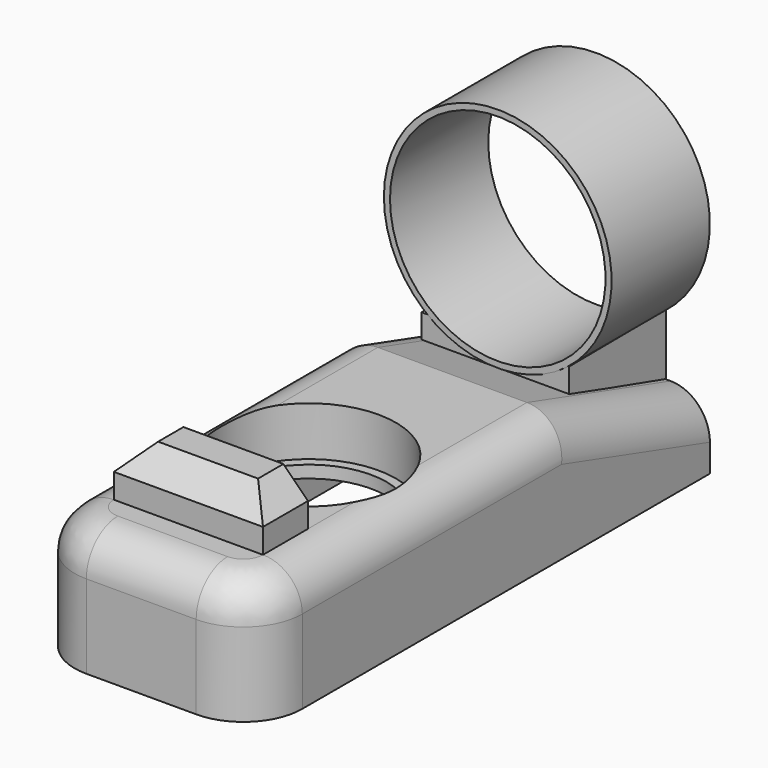
from build123d import *

# Parameters (mm, degrees)
F0_W           = 46.3467240334
F0_H           = 115.6897172332
F1_DEPTH       = 25
F2_R           = 12
F4_DEPTH       = 40
F4_DEPTH_BACK  = 40
F6_R           = 17.7712313218
F7_DEPTH       = 10
F8_R           = 23.1733620167
F9_DEPTH       = 25
F11_R          = 21.9307918762
F12_DEPTH      = 25
F14_DEPTH      = 15
F14_DEPTH_BACK = 15
F15_T          = 2.5
F16_R          = 15.8642477534
F17_DEPTH      = 25
F18_DEPTH      = 5
F19_DEPTH      = 25
F20_T1_DEPTH   = 101.1275982577
F20_T3_DEPTH   = 92.184276345
F20_T5_DEPTH   = 22.3467240334
F20_T8_ANGLE   = 90
F20_T12_DEPTH  = 92.184276345
F20_T17_DEPTH  = 92.184276345
F20_T22_DEPTH  = 92.184276345
F20_T27_DEPTH  = 101.1275982577
F20_T30_ANGLE  = 90
F21_W          = 30.3467240334
F21_H          = 11.4395302832
F22_DEPTH      = 10
F23_SIZE       = 5


# Not quite as in the source:
# - a fillet or chamfer that OpenCascade refuses, or shapes differently, is made with other operations: its cross-section is extruded or revolved along the edge and cut away or added
# - a shell that OpenCascade refuses in one call is made with other operations: the cavity is built on its own and cut out


with BuildPart() as f1:
    # F0 (on Top) → F1 (new body)
    with BuildSketch(Plane.XY):
        with Locations((7.814258337, 1.8636099994)):
            Rectangle(F0_W, F0_H)
    extrude(amount=F1_DEPTH)

    # F2
    f2_edges = [f1.edges().sort_by_distance(p)[0] for p in [
        (30.98762, -55.981249, 12.5),
        (-15.359104, -55.981249, 12.5),
    ]]
    fillet(f2_edges, radius=F2_R)

    # F3 (on Right) → F4 (cut, two sides)
    with BuildSketch(Plane.YZ) as f4_sk:
        Polygon((0, 31.970962882), (68.2880878448, 11.4047080278), (67.6364898682, 28.4685865045), align=None)
    extrude(amount=F4_DEPTH, mode=Mode.SUBTRACT)
    extrude(f4_sk.sketch, amount=-F4_DEPTH_BACK, mode=Mode.SUBTRACT)


with BuildPart() as f1_1:
    # F5: moved
    add(f1.part.moved(Location((-7.1676671505, 0, 0))))

    # F6 (on face) → F7 (cut)
    with BuildSketch(Plane.XY.offset(25)):
        with Locations((0, -12.5934332609)):
            Circle(F6_R)
    extrude(amount=-F7_DEPTH, mode=Mode.SUBTRACT)

    # F15: shell of thickness 2.5, made by hand


with BuildPart() as f9:
    # F8 (on face) → F9 (new body)
    with BuildSketch(Plane(origin=(0, 59.708468616, 0), x_dir=(-1, 0, 0), z_dir=(0, 1, 0))):
        with Locations((-0.6465911865, 33.9257717133)):
            Circle(F8_R)
    extrude(amount=-F9_DEPTH)


with BuildPart() as f9_1:
    # F10: moved
    add(f9.part.moved(Location((0, 0, 10.7776373625))))

    # F11 (on face) → F12 (cut)
    with BuildSketch(Plane(origin=(0, 59.708468616, 0), x_dir=(-1, 0, 0), z_dir=(0, 1, 0))):
        with Locations((-0.6465911865, 44.7034090757)):
            Circle(F11_R)
    extrude(amount=-F12_DEPTH, mode=Mode.SUBTRACT)


with BuildPart() as f14:
    # F13 (on Right) → F14 (new body, two sides)
    with BuildSketch(Plane.YZ) as f14_sk:
        Polygon((59.624966234, 14.1331925988), (59.624966234, 21.5853508562), (34.9215567112, 21.3780961931), align=None)
    extrude(amount=F14_DEPTH)
    extrude(f14_sk.sketch, amount=-F14_DEPTH_BACK)


with BuildPart() as f15_core1:
    # F15_t2: copy of F1
    add(f1_1.part)

    # the walls: a layer under each face that stays
    f15_faces = [f15_core1.faces().sort_by_distance(p)[0] for p in [
        (-22.5267708302, 7.8636099994, 12.5),
        (-19.0120522044, -52.4665299914, 12.5),
        (-14.8023168246, -42.7933155742, 25),
        (0.6465911865, 41.4274091283, 19.4943116685),
        (0.6465911865, 59.708468616, 6.9943116685),
        (0.6465911865, -55.9812486172, 12.5),
        (23.8199532032, 7.8636099994, 12.5),
        (20.3052345774, -52.4665299914, 12.5),
        (-17.7712313218, -12.5934332609, 20),
        (0, -12.5934332609, 15),
    ]]
    thicken(f15_faces, amount=-F15_T, mode=Mode.SUBTRACT)

    # F15_s3 → F15_t4 (revolve, cut)
    with BuildSketch(Plane.XZ.offset(12.5934332609)):
        Polygon((17.7462313218, 15.025), (20.2712313218, 15), (20.2712313218, 12.5), (17.7712313218, 12.5), align=None)
    revolve(axis=Axis((0, -12.5934332609, 15), (0, 0, 1)), mode=Mode.SUBTRACT)


with BuildPart() as f1_2:
    add(f1_1.part)

    # what is left inside the walls is the cavity
    f15_cavity = [f15_core1.part.solids().sort_by_distance(p)[0] for p in [
        (0.646591, -16.584676, 0.025),
    ]]
    add(f15_cavity, mode=Mode.SUBTRACT)

    # F16 (on face) → F17 (cut)
    with BuildSketch(Plane.XY.offset(15)):
        with Locations((0, -12.5934332609)):
            Circle(F16_R)
    extrude(amount=-F17_DEPTH, mode=Mode.SUBTRACT)

    # F18 (add): a face of the model
    f18_faces = [f14.part.faces().sort_by_distance(p)[0] for p in [
        (0, 47.2732614726, 21.4817235246),
    ]]

    add(f9_1.part)  # F18 merges F9

    add(f14.part)  # F18 merges F14
    extrude(f18_faces, amount=F18_DEPTH)

    # F11 (on face) → F19 (cut)
    with BuildSketch(Plane(origin=(0, 59.708468616, 0), x_dir=(-1, 0, 0), z_dir=(0, 1, 0))):
        with Locations((-0.6465911865, 44.7034090757)):
            Circle(F11_R)
    extrude(amount=-F19_DEPTH, mode=Mode.SUBTRACT)

    # F20: fillet of radius 8 on 7 edges, made by hand

    # F20_s2 → F20_t1 (cut)
    with BuildSketch(Plane.XZ.offset(-57.1463496406)):
        with BuildLine():
            ThreePointArc((15.8199532032, 25), (21.4768074527, 22.6568542495), (23.8199532032, 17))
            Line((23.8199532032, 17), (23.8199532032, 25))
            Line((23.8199532032, 25), (15.8199532032, 25))
        make_face()
    extrude(amount=F20_T1_DEPTH, mode=Mode.SUBTRACT)

    # F20_s4 → F20_t3 (cut)
    with BuildSketch(Plane(origin=(0, -18.2371947161, 5.4924776223), x_dir=(1, 0, 0), z_dir=(0, 0.9575176611, -0.2883746326))):
        with BuildLine():
            ThreePointArc((15.8199532032, -30.6127616009), (21.4768074527, -28.2696158504), (23.8199532032, -22.6127616009))
            Line((23.8199532032, -22.6127616009), (23.8199532032, -30.6127616009))
            Line((23.8199532032, -30.6127616009), (15.8199532032, -30.6127616009))
        make_face()
    extrude(amount=F20_T3_DEPTH, mode=Mode.SUBTRACT)

    # F20_s6 → F20_t5 (cut)
    with BuildSketch(Plane.YZ.offset(-10.5267708302)):
        with BuildLine():
            ThreePointArc((-47.9812486172, 25), (-53.6381028667, 22.6568542495), (-55.9812486172, 17))
            Line((-55.9812486172, 17), (-55.9812486172, 25))
            Line((-55.9812486172, 25), (-47.9812486172, 25))
        make_face()
    extrude(amount=F20_T5_DEPTH, mode=Mode.SUBTRACT)

    # F20_s7 → F20_t8 (revolve, cut)
    with BuildSketch(Plane.YZ.offset(11.8199532032)):
        with BuildLine():
            ThreePointArc((-47.9812486172, 25), (-53.6381028667, 22.6568542495), (-55.9812486172, 17))
            Line((-55.9812486172, 17), (-55.9812486172, 25))
            Line((-55.9812486172, 25), (-47.9812486172, 25))
        make_face()
    revolve(axis=Axis((11.8199532032, -43.9812486172, 25), (0, 0, 1)), revolution_arc=F20_T8_ANGLE, mode=Mode.SUBTRACT)


with BuildPart() as f20_tool10:
    # F20_s11 → F20_t12 (new body)
    with BuildSketch(Plane(origin=(0, 70.0308779571, -21.0911292025), x_dir=(1, 0, 0), z_dir=(0, -0.9575176611, 0.2883746326))):
        with BuildLine():
            ThreePointArc((-14.5267708302, 30.6127616009), (-20.1836250796, 28.2696158504), (-22.5267708302, 22.6127616009))
            Line((-22.5267708302, 22.6127616009), (-22.5267708302, 30.6127616009))
            Line((-22.5267708302, 30.6127616009), (-14.5267708302, 30.6127616009))
        make_face()
    extrude(amount=F20_T12_DEPTH)

    split(bisect_by=Plane(origin=(0, 8.5388595544, 29.1154936273), x_dir=(1, 0, 0), z_dir=(0, -0.281422426, -0.9595839818)), keep=Keep.TOP)


with BuildPart() as f1_3:
    add(f1_2.part)

    # F20_t9: cut F20_tool10
    add(f20_tool10.part, mode=Mode.SUBTRACT)


with BuildPart() as f20_tool15:
    # F20_s16 → F20_t17 (new body)
    with BuildSketch(Plane(origin=(0, 70.0308779571, -21.0911292025), x_dir=(1, 0, 0), z_dir=(0, -0.9575176611, 0.2883746326))):
        with BuildLine():
            ThreePointArc((-14.5267708302, 30.6127616009), (-20.1836250796, 28.2696158504), (-22.5267708302, 22.6127616009))
            Line((-22.5267708302, 22.6127616009), (-22.5267708302, 30.6127616009))
            Line((-22.5267708302, 30.6127616009), (-14.5267708302, 30.6127616009))
        make_face()
    extrude(amount=F20_T17_DEPTH)

    split(bisect_by=Plane.YZ.offset(-15), keep=Keep.BOTTOM)


with BuildPart() as f1_4:
    add(f1_3.part)

    # F20_t14: cut F20_tool15
    add(f20_tool15.part, mode=Mode.SUBTRACT)


with BuildPart() as f20_tool20:
    # F20_s21 → F20_t22 (new body)
    with BuildSketch(Plane(origin=(0, 70.0308779571, -21.0911292025), x_dir=(1, 0, 0), z_dir=(0, -0.9575176611, 0.2883746326))):
        with BuildLine():
            ThreePointArc((-14.5267708302, 30.6127616009), (-20.1836250796, 28.2696158504), (-22.5267708302, 22.6127616009))
            Line((-22.5267708302, 22.6127616009), (-22.5267708302, 30.6127616009))
            Line((-22.5267708302, 30.6127616009), (-14.5267708302, 30.6127616009))
        make_face()
    extrude(amount=F20_T22_DEPTH)

    split(bisect_by=Plane(origin=(0, 35.0984424425, 0.2944660678), x_dir=(1, 0, 0), z_dir=(0, -0.9999648082, -0.0083894237)), keep=Keep.TOP)


with BuildPart() as f1_5:
    add(f1_4.part)

    # F20_t19: cut F20_tool20
    add(f20_tool20.part, mode=Mode.SUBTRACT)


with BuildPart() as f20_tool25:
    # F20_s26 → F20_t27 (new body)
    with BuildSketch(Plane.XZ.offset(-57.1463496406)):
        with BuildLine():
            ThreePointArc((-22.5267708302, 17), (-20.1836250796, 22.6568542495), (-14.5267708302, 25))
            Line((-14.5267708302, 25), (-22.5267708302, 25))
            Line((-22.5267708302, 25), (-22.5267708302, 17))
        make_face()
    extrude(amount=F20_T27_DEPTH)

    split(bisect_by=Plane(origin=(0, 8.8279438803, 29.312259887), x_dir=(1, 0, 0), z_dir=(0, -0.2883746326, -0.9575176611)), keep=Keep.TOP)


with BuildPart() as f1_6:
    add(f1_5.part)

    # F20_t24: cut F20_tool25
    add(f20_tool25.part, mode=Mode.SUBTRACT)

    # F20_s29 → F20_t30 (revolve, cut)
    with BuildSketch(Plane.XZ.offset(43.9812486172)):
        with BuildLine():
            ThreePointArc((-14.5267708302, 25), (-20.1836250796, 22.6568542495), (-22.5267708302, 17))
            Line((-22.5267708302, 17), (-22.5267708302, 25))
            Line((-22.5267708302, 25), (-14.5267708302, 25))
        make_face()
    revolve(axis=Axis((-10.5267708302, -43.9812486172, 25), (0, 0, 1)), revolution_arc=F20_T30_ANGLE, mode=Mode.SUBTRACT)

    # F21 (on face) → F22 (join)
    with BuildSketch(Plane.XY.offset(25)):
        with Locations((0.6465911865, -38.2614834756)):
            Rectangle(F21_W, F21_H)
    extrude(amount=F22_DEPTH)

    # F23
    f23_edges = [f1_6.edges().sort_by_distance(p)[0] for p in [
        (15.819953, -38.261483, 35),
        (-14.526771, -38.261483, 35),
        (0.646591, -43.981249, 35),
    ]]
    chamfer(f23_edges, length=F23_SIZE)


solid = f1_6.part
